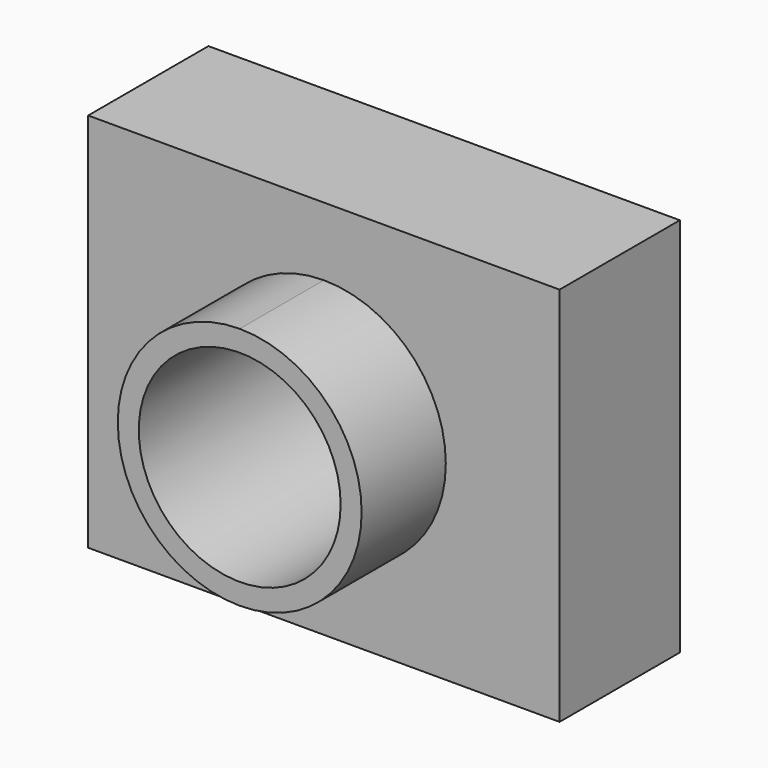
from build123d import *

# Parameters (mm, degrees)
F0_W     = 79.6634554863
F0_H     = 64.3117427826
F0_R     = 20.6041591681
F1_DEPTH = 25.4
F3_DEPTH = 43.18
F4_R     = 17.0569002262
F5_DEPTH = 50.8


with BuildPart() as f1:
    # F0 (on Front) → F1 (new body)
    with BuildSketch(Plane.XZ):
        Rectangle(F0_W, F0_H)
        Circle(F0_R, mode=Mode.SUBTRACT)
    extrude(amount=F1_DEPTH)


with BuildPart() as f3:
    # F2 (on face) → F3 (new body)
    with BuildSketch(Plane(origin=(0, 0, 0), x_dir=(-1, 0, 0), z_dir=(0, 1, 0))):
        with BuildLine():
            ThreePointArc((0, -20.6041591681), (14.5693406684, -14.5693406684), (20.6041591681, 0))
            ThreePointArc((20.6041591681, 0), (14.5693406684, 14.5693406684), (0, 20.6041591681))
            ThreePointArc((0, 20.6041591681), (-20.6041591681, 0), (0, -20.6041591681))
        make_face()
    extrude(amount=-F3_DEPTH)

    # F4 (on face) → F5 (cut)
    with BuildSketch(Plane.XZ.offset(43.18)):
        Circle(F4_R)
    extrude(amount=-F5_DEPTH, mode=Mode.SUBTRACT)


solid = Compound([f1.part, f3.part])
